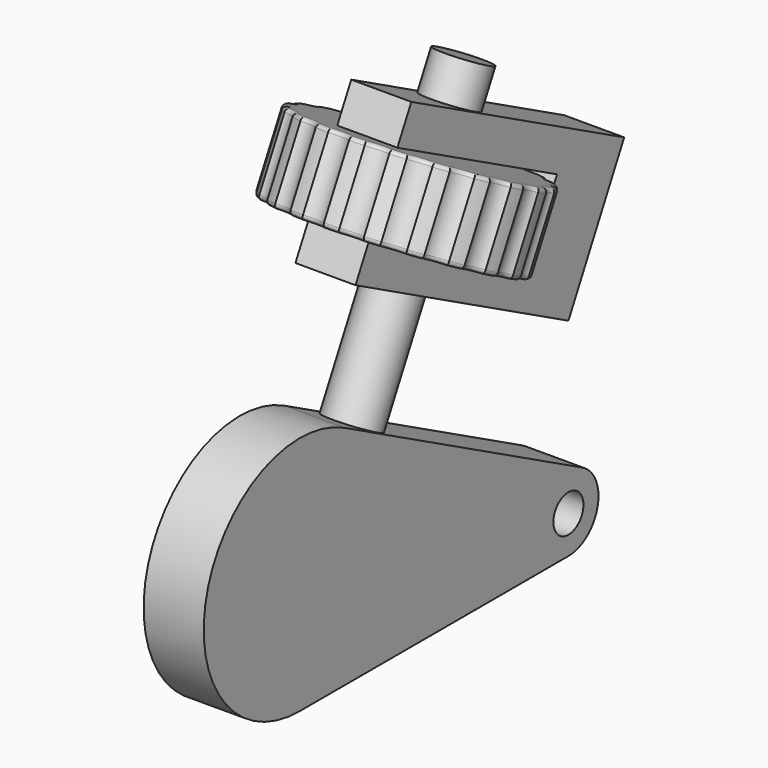
from build123d import *

# Parameters (mm, degrees)
F0_R     = 2.5
F1_DEPTH = 8
F2_R     = 3.5
F3_DEPTH = 40
F5_DEPTH = 8
F6_R     = 3.5
F7_DEPTH = 10
F8_R     = 0.5


with BuildPart() as f1:
    # F0 (on Right) → F1 (new body)
    with BuildSketch(Plane.YZ):
        with BuildLine():
            ThreePointArc((0, -16), (11.313708499, -11.313708499), (16, 0))
            ThreePointArc((16, 0), (13.6899711133, 8.2815874636), (7.4269136353, 14.1718366436))
            ThreePointArc((7.4269136353, 14.1718366436), (-15.536238063, 3.824304754), (0, -16))
        make_face()
        with BuildLine():
            ThreePointArc((7.4269136353, 14.1718366436), (13.6899711133, 8.2815874636), (16, 0))
            ThreePointArc((16, 0), (11.313708499, -11.313708499), (0, -16))
            Line((0, -16), (35.457721303, -16))
            ThreePointArc((35.457721303, -16), (34.6241715475, -15.552444391), (34.5367415289, -14.6103896104))
            ThreePointArc((34.5367415289, -14.6103896104), (35.9177848654, -10.777881534), (36.8749562263, -6.8181818182))
            ThreePointArc((36.8749562263, -6.8181818182), (37.2186862433, -6.2312938852), (37.8582883924, -6))
            Line((37.8582883924, -6), (40.215364045, -6))
            ThreePointArc((40.215364045, -6), (41.1282349742, -6.5917517095), (40.9607200375, -7.6666666667))
            ThreePointArc((40.9607200375, -7.6666666667), (39.6875, -11), (40.9607200375, -14.3333333333))
            ThreePointArc((40.9607200375, -14.3333333333), (41.1282349742, -15.4082482905), (40.215364045, -16))
            Line((40.215364045, -16), (44.6875, -16))
            ThreePointArc((44.6875, -16), (49.5425743947, -12.1950952356), (47.008410511, -6.5713010489))
            Line((47.008410511, -6.5713010489), (7.4269136353, 14.1718366436))
        make_face()
        with Locations((44.6875, -11)):
            Circle(F0_R, mode=Mode.SUBTRACT)
        with BuildLine():
            ThreePointArc((34.5367415289, -14.6103896104), (34.6241715475, -15.552444391), (35.457721303, -16))
            Line((35.457721303, -16), (40.215364045, -16))
            ThreePointArc((40.215364045, -16), (41.1282349742, -15.4082482905), (40.9607200375, -14.3333333333))
            ThreePointArc((40.9607200375, -14.3333333333), (39.6875, -11), (40.9607200375, -7.6666666667))
            ThreePointArc((40.9607200375, -7.6666666667), (41.1282349742, -6.5917517095), (40.215364045, -6))
            Line((40.215364045, -6), (37.8582883924, -6))
            ThreePointArc((37.8582883924, -6), (37.2186862433, -6.2312938852), (36.8749562263, -6.8181818182))
            ThreePointArc((36.8749562263, -6.8181818182), (35.9177848654, -10.777881534), (34.5367415289, -14.6103896104))
        make_face()
    extrude(amount=F1_DEPTH)


with BuildPart() as f3:
    # F2 (on face) → F3 (new body)
    with BuildSketch(Plane(origin=(0, 7.4269136353, 14.1718366436), x_dir=(1, 0, 0), z_dir=(0, 0.4641821022, 0.8857397902))):
        with Locations((4, 7)):
            Circle(F2_R)
    extrude(amount=F3_DEPTH)


with BuildPart() as f5:
    # F4 (on Right) → F5 (new body)
    with BuildSketch(Plane.YZ):
        Polygon((11.578818902, 34.5759780004), (9.257908391, 30.1472790493), (44.6875, 11.5799949609), (53.9711420442, 29.2947907655), (18.5415504352, 47.8620748538), (16.2206399241, 43.4333759027), (42.7928336309, 29.5079128364), (38.1510126088, 20.6505149342), align=None)
    extrude(amount=F5_DEPTH)


with BuildPart() as f7:
    # F6 (on face) → F7 (new body)
    with BuildSketch(Plane(origin=(0, 16.7105556795, 31.8866324481), x_dir=(1, 0, 0), z_dir=(0, 0.4641821022, 0.8857397902))):
        with BuildLine():
            ThreePointArc((18.9193672131, 2.6530538213), (18.4992020588, 4.0648090065), (18.9468321871, 5.4680975471))
            ThreePointArc((18.9468321871, 5.4680975471), (18.8375127324, 6.408136933), (18.6691317478, 7.3394116692))
            ThreePointArc((18.6691317478, 7.3394116692), (17.8332745958, 8.5522324645), (17.8253561391, 10.0251644921))
            ThreePointArc((17.8253561391, 10.0251644921), (17.4308990137, 10.8854135063), (16.9829794611, 11.7190758268))
            ThreePointArc((16.9829794611, 11.7190758268), (15.8132498332, 12.6142428824), (15.3505579053, 14.0126375477))
            ThreePointArc((15.3505579053, 14.0126375477), (14.709575321, 14.708889023), (14.0259626871, 15.3633342514))
            ThreePointArc((14.0259626871, 15.3633342514), (12.6368618691, 15.8532223789), (11.7646879797, 17.0401950688))
            ThreePointArc((11.7646879797, 17.0401950688), (10.9399237778, 17.5042950597), (10.0875348303, 17.9154615374))
            ThreePointArc((10.0875348303, 17.9154615374), (9.0057309593, 17.8551328076), (8, 18.2581767361))
            Line((8, 18.2581767361), (8, -5.7937295288))
            Line((8, -5.7937295288), (0, -5.7937295288))
            Line((0, -5.7937295288), (0, 18.1773049578))
            ThreePointArc((0, 18.1773049578), (-0.8956811946, 17.9325901376), (-1.8188940209, 18.0316266103))
            ThreePointArc((-1.8188940209, 18.0316266103), (-2.6791430351, 17.6371694848), (-3.5128053557, 17.1892499323))
            ThreePointArc((-3.5128053557, 17.1892499323), (-4.4079724113, 16.0195203043), (-5.8063670765, 15.5568283764))
            ThreePointArc((-5.8063670765, 15.5568283764), (-6.5026185518, 14.9158457921), (-7.1570637803, 14.2322331582))
            ThreePointArc((-7.1570637803, 14.2322331582), (-7.6469519078, 12.8431323403), (-8.8339245977, 11.9709584508))
            ThreePointArc((-8.8339245977, 11.9709584508), (-9.2980245886, 11.146194249), (-9.7091910662, 10.2938053014))
            ThreePointArc((-9.7091910662, 10.2938053014), (-9.6392860707, 9.958611755), (-9.6158377863, 9.6170102328))
            ThreePointArc((-9.6158377863, 9.6170102328), (-9.8768007091, 8.504934261), (-10.60520816, 7.625026766))
            ThreePointArc((-10.60520816, 7.625026766), (-10.7917273258, 6.6972146131), (-10.9193672131, 5.759487121))
            ThreePointArc((-10.9193672131, 5.759487121), (-10.6064600777, 5.0969359082), (-10.4990830807, 4.3721220249))
            ThreePointArc((-10.4990830807, 4.3721220249), (-10.6136452557, 3.6240001211), (-10.9468321871, 2.9444433952))
            ThreePointArc((-10.9468321871, 2.9444433952), (-10.8375127324, 2.0044040093), (-10.6691317478, 1.0731292731))
            ThreePointArc((-10.6691317478, 1.0731292731), (-9.9685597122, 0.2011780326), (-9.7183396836, -0.8890008886))
            ThreePointArc((-9.7183396836, -0.8890008886), (-9.7452385068, -1.2547474804), (-9.8253561391, -1.6126235498))
            ThreePointArc((-9.8253561391, -1.6126235498), (-9.4308990137, -2.472872564), (-8.9829794611, -3.3065348845))
            ThreePointArc((-8.9829794611, -3.3065348845), (-7.8132498332, -4.2017019401), (-7.3505579053, -5.6000966054))
            ThreePointArc((-7.3505579053, -5.6000966054), (-6.709575321, -6.2963480807), (-6.0259626871, -6.9507933091))
            ThreePointArc((-6.0259626871, -6.9507933091), (-4.6368618691, -7.4406814366), (-3.7646879797, -8.6276541265))
            ThreePointArc((-3.7646879797, -8.6276541265), (-2.9399237778, -9.0917541174), (-2.0875348303, -9.5029205951))
            ThreePointArc((-2.0875348303, -9.5029205951), (-0.6150376888, -9.5395761314), (0.5812437051, -10.3989376888))
            ThreePointArc((0.5812437051, -10.3989376888), (1.509055858, -10.5854568547), (2.4467833501, -10.7130967419))
            ThreePointArc((2.4467833501, -10.7130967419), (3.8585385354, -10.2929315877), (5.261827076, -10.740561716))
            ThreePointArc((5.261827076, -10.740561716), (6.2018664619, -10.6312422612), (7.1331411981, -10.4628612766))
            ThreePointArc((7.1331411981, -10.4628612766), (8.3459619933, -9.6270041246), (9.8188940209, -9.619085668))
            ThreePointArc((9.8188940209, -9.619085668), (10.6791430351, -9.2246285425), (11.5128053557, -8.77670899))
            ThreePointArc((11.5128053557, -8.77670899), (12.4079724113, -7.606979362), (13.8063670765, -7.1442874341))
            ThreePointArc((13.8063670765, -7.1442874341), (14.5026185518, -6.5033048498), (15.1570637803, -5.8196922159))
            ThreePointArc((15.1570637803, -5.8196922159), (15.6469519078, -4.430591398), (16.8339245977, -3.5584175085))
            ThreePointArc((16.8339245977, -3.5584175085), (17.2980245886, -2.7336533067), (17.7091910662, -1.8812643591))
            ThreePointArc((17.7091910662, -1.8812643591), (17.7458466025, -0.4087672176), (18.60520816, 0.7875141763))
            ThreePointArc((18.60520816, 0.7875141763), (18.7917273258, 1.7153263292), (18.9193672131, 2.6530538213))
        make_face()
        with BuildLine():
            Line((8, -5.7937295288), (8, 18.2581767361))
            ThreePointArc((8, 18.2581767361), (7.6870323941, 18.5113534671), (7.4187562949, 18.8114786311))
            ThreePointArc((7.4187562949, 18.8114786311), (6.490944142, 18.997997797), (5.5532166499, 19.1256376842))
            ThreePointArc((5.5532166499, 19.1256376842), (4.1414614646, 18.70547253), (2.738172924, 19.1531026583))
            ThreePointArc((2.738172924, 19.1531026583), (1.7981335381, 19.0437832035), (0.8668588019, 18.8754022189))
            ThreePointArc((0.8668588019, 18.8754022189), (0.4727723138, 18.4774997219), (0, 18.1773049578))
            Line((0, 18.1773049578), (0, -5.7937295288))
            Line((0, -5.7937295288), (8, -5.7937295288))
        make_face()
        with Locations((4, 4.2062704712)):
            Circle(F6_R, mode=Mode.SUBTRACT)
    extrude(amount=F7_DEPTH)

    # F8
    f8_edges = [f7.edges().sort_by_distance(p)[0] for p in [
        (12.407972, 14.614572, 44.275054),
        (14.502619, 15.592141, 43.762748),
        (15.646952, 17.428026, 42.800632),
        (17.298025, 18.931071, 42.012943),
        (17.745847, 20.990315, 40.933773),
        (18.791727, 22.871709, 39.947807),
        (18.499202, 24.95274, 38.857219),
        (18.837513, 27.028319, 37.769488),
        (17.833275, 28.927429, 36.774237),
        (17.430899, 30.994021, 35.691216),
        (15.81325, 32.525314, 34.888725),
        (14.709575, 34.380625, 33.916427),
        (12.636862, 35.394207, 33.385248),
        (10.939924, 36.856627, 32.61885),
        (8.615038, 37.253281, 32.410979),
        (6.490944, 38.179659, 31.9255),
        (4.141461, 37.920558, 32.061285),
        (1.798134, 38.220213, 31.904247),
        (-0.345962, 37.33072, 32.370396),
        (-2.679143, 36.97432, 32.557172),
        (-4.407972, 35.541503, 33.308056),
        (-6.502619, 34.563935, 33.820362),
        (-7.646952, 32.72805, 34.782478),
        (-9.298025, 31.225004, 35.570166),
        (-9.745847, 29.16576, 36.649337),
        (-10.791727, 27.284366, 37.635303),
        (-10.499202, 25.203336, 38.725891),
        (-10.837513, 23.127757, 39.813622),
        (-9.833275, 21.228646, 40.808873),
        (-9.430899, 19.162055, 41.891894),
        (-7.81325, 17.630762, 42.694385),
        (-6.709575, 15.775451, 43.666682),
        (-4.636862, 14.761869, 44.197862),
        (-2.939924, 13.299448, 44.96426),
        (-0.615038, 12.902795, 45.172131),
        (1.509056, 11.976416, 45.65761),
        (3.858539, 12.235518, 45.521825),
        (6.201866, 11.935862, 45.678863),
        (8.345962, 12.825356, 45.212713),
        (10.679143, 13.181756, 45.025938),
        (0.5, 25.078038, 38.791555),
        (12.407972, 9.972751, 35.417656),
        (14.502619, 10.95032, 34.90535),
        (15.646952, 12.786205, 33.943234),
        (17.298025, 14.28925, 33.155545),
        (17.745847, 16.348494, 32.076375),
        (18.791727, 18.229888, 31.090409),
        (18.499202, 20.310919, 29.999821),
        (18.837513, 22.386498, 28.91209),
        (17.833275, 24.285608, 27.916839),
        (17.430899, 26.3522, 26.833818),
        (15.81325, 27.883493, 26.031327),
        (14.709575, 29.738804, 25.059029),
        (12.636862, 30.752386, 24.52785),
        (10.939924, 32.214806, 23.761452),
        (8.615038, 32.61146, 23.553581),
        (6.490944, 33.537838, 23.068102),
        (4.141461, 33.278737, 23.203887),
        (1.798134, 33.578392, 23.046849),
        (-0.345962, 32.688899, 23.512998),
        (-2.679143, 32.332498, 23.699774),
        (-4.407972, 30.899682, 24.450658),
        (-6.502619, 29.922114, 24.962964),
        (-7.646952, 28.086229, 25.92508),
        (-9.298025, 26.583183, 26.712769),
        (-9.745847, 24.523939, 27.791939),
        (-10.791727, 22.642545, 28.777905),
        (-10.499202, 20.561515, 29.868493),
        (-10.837513, 18.485936, 30.956224),
        (-9.833275, 16.586825, 31.951475),
        (-9.430899, 14.520234, 33.034496),
        (-7.81325, 12.988941, 33.836987),
        (-6.709575, 11.13363, 34.809285),
        (-4.636862, 10.120048, 35.340464),
        (-2.939924, 8.657627, 36.106862),
        (-0.615038, 8.260974, 36.314733),
        (1.509056, 7.334595, 36.800212),
        (3.858539, 7.593697, 36.664427),
        (6.201866, 7.294041, 36.821465),
        (8.345962, 8.183535, 36.355315),
        (10.679143, 8.539935, 36.16854),
        (0.5, 20.436217, 29.934157),
    ]]
    fillet(f8_edges, radius=F8_R)


solid = Compound([f1.part, f3.part, f5.part, f7.part])
